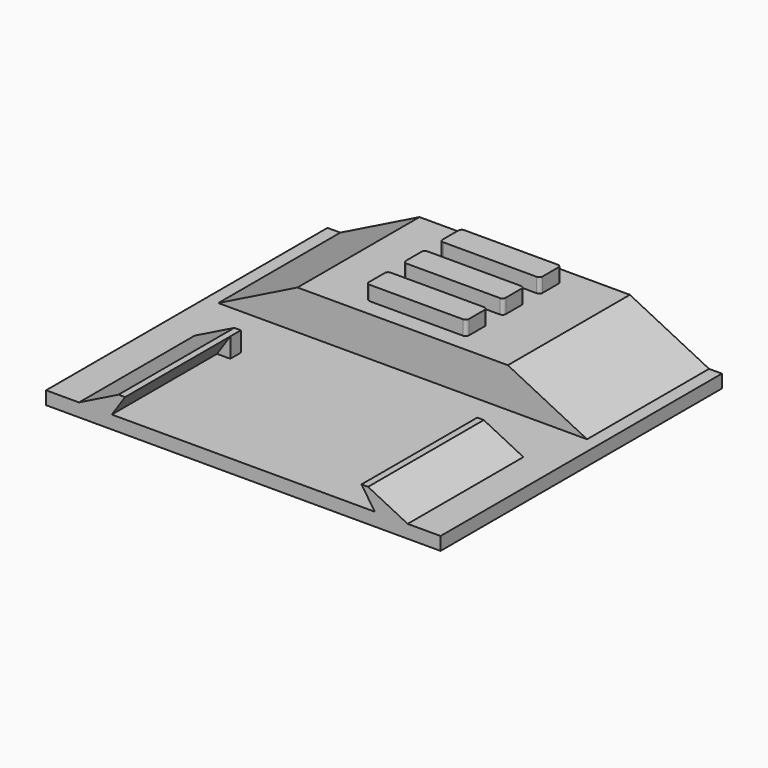
from build123d import *

# Parameters (mm, degrees)
F0_W      = 60
F0_H      = 53.5
F1_DEPTH  = 2
F3_DEPTH  = 23.2
F4_W      = 15.2
F4_H      = 4
F5_DEPTH  = 2.2
F6_R      = 0.5
F8_DEPTH  = 20
F11_DEPTH = 2


with BuildPart() as f1:
    # F0 (on Top) → F1 (new body)
    with BuildSketch(Plane.XY):
        with Locations((30, 26.75)):
            Rectangle(F0_W, F0_H)
    extrude(amount=F1_DEPTH)

    # F2 (on face) → F3 (join)
    with BuildSketch(Plane(origin=(0, 53.5, 0), x_dir=(-1, 0, 0), z_dir=(0, 1, 0))):
        Polygon((-1.9529488989, 2), (-14, 8), (-46, 8), (-58.0470511011, 2), align=None)
    extrude(amount=-F3_DEPTH)

    # F4 (on face) → F5 (join)
    with BuildSketch(Plane.XY.offset(8)):
        with Locations((30, 48.9)):
            Rectangle(F4_W, F4_H)
        with Locations((30, 41.9)):
            Rectangle(F4_W, F4_H)
        with Locations((30, 34.9)):
            Rectangle(F4_W, F4_H)
    extrude(amount=F5_DEPTH)

    # F6
    f6_edges = [f1.edges().sort_by_distance(p)[0] for p in [
        (22.4, 46.9, 9.1),
        (22.4, 39.9, 9.1),
        (22.4, 32.9, 9.1),
        (22.4, 36.9, 9.1),
        (22.4, 43.9, 9.1),
        (22.4, 50.9, 9.1),
        (37.6, 32.9, 9.1),
        (37.6, 36.9, 9.1),
        (37.6, 39.9, 9.1),
        (37.6, 43.9, 9.1),
        (37.6, 46.9, 9.1),
        (37.6, 50.9, 9.1),
    ]]
    fillet(f6_edges, radius=F6_R)

    # F7 (on face) → F8 (join)
    with BuildSketch(Plane.XZ):
        Polygon((5, 2), (10, 2), (12.0235255505, 5), (11.0235255505, 5), align=None)
        Polygon((47.9764744495, 5), (50, 2), (55, 2), (48.9764744495, 5), align=None)
    extrude(amount=-F8_DEPTH)

    # F9 (on face) + F10 (on face) → F11 (join)
    with BuildSketch(Plane(origin=(0, 20, 0), x_dir=(-1, 0, 0), z_dir=(0, 1, 0))):
        Polygon((-10, 2), (-5, 2), (-11.0235255505, 5), (-12.0235255505, 5), align=None)
        Polygon((-12.0235255505, 2), (-10, 2), (-12.0235255505, 5), align=None)
    with BuildSketch(Plane(origin=(0, 20, 0), x_dir=(-1, 0, 0), z_dir=(0, 1, 0))):
        Polygon((-47.9764744495, 5), (-50, 2), (-47.9764744495, 2), align=None)
        Polygon((-48.9764744495, 5), (-55, 2), (-50, 2), (-47.9764744495, 5), align=None)
    extrude(amount=F11_DEPTH)


solid = f1.part
